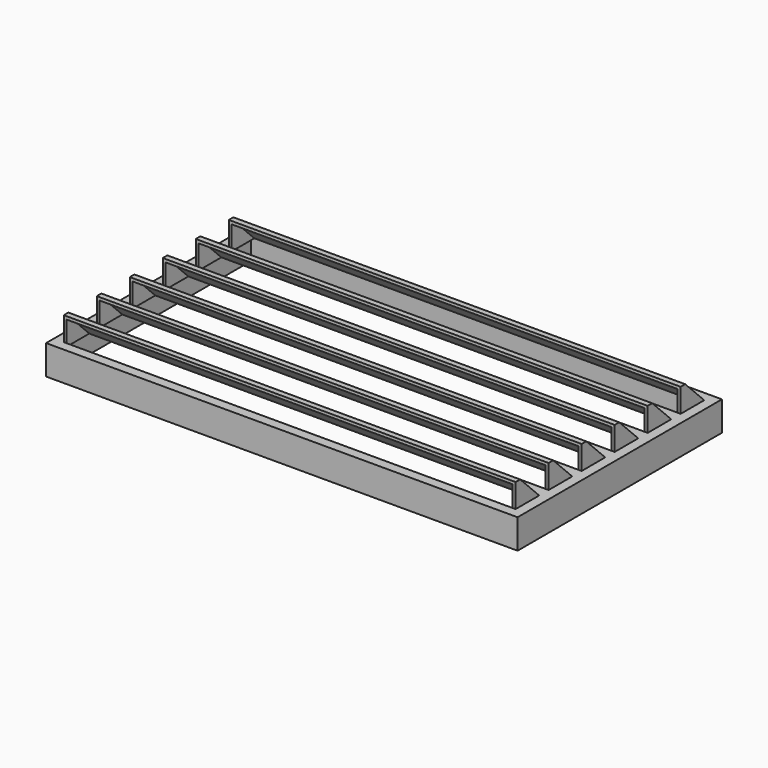
from build123d import *

# Parameters (mm, degrees)
F0_W         = 1200
F0_H         = 650
F1_DEPTH     = 75
F3_START     = -25
F3_DEPTH     = 1150
F4_T         = 7.5
F4_T3_DEPTH  = 90
F4_T5_DEPTH  = 1165
F4_T7_DEPTH  = 90
F4_T9_DEPTH  = 90
F4_T11_DEPTH = 90
F4_T13_DEPTH = 90
F4_T15_DEPTH = 90


# Not quite as in the source:
# - a shell that OpenCascade refuses in one call is made with other operations: the cavity is built on its own and cut out
# - a feature names something its author has since deleted; it is built from what else it names


with BuildPart() as f1:
    # F0 (on Top) → F1 (new body)
    with BuildSketch(Plane.XY):
        Rectangle(F0_W, F0_H)
    extrude(amount=F1_DEPTH)

    # F2 (on face) → F3 (join)
    with BuildSketch(Plane(origin=(-600, 0, 0), x_dir=(0, -1, 0), z_dir=(-1, 0, 0)).offset(F3_START)):
        Polygon((-239.4699645042, 135.5300354958), (-300, 75), (-225, 75), (-225, 135.5300354958), align=None)
        Polygon((-134.4699645042, 135.5300354958), (-195, 75), (-120, 75), (-120, 135.5300354958), align=None)
        Polygon((-29.4699645042, 135.5300354958), (-90, 75), (-15, 75), (-15, 135.5300354958), align=None)
        Polygon((75.5300354958, 135.5300354958), (15, 75), (90, 75), (90, 135.5300354958), align=None)
        Polygon((120, 75), (195, 75), (195, 135.5300354958), (180.5300354958, 135.5300354958), align=None)
        Polygon((225, 75), (300, 75), (300, 135.5300354958), (285.5300354958, 135.5300354958), align=None)
    extrude(amount=-F3_DEPTH)

    # F4: shell of thickness 7.5, made by hand


with BuildPart() as f4_core1:
    # F4_t2: copy of F1
    add(f1.part)

    # the walls: a layer under each face that stays
    f4_faces = [f4_core1.faces().sort_by_distance(p)[0] for p in [
        (0, -325, 37.5),
        (-600, 0, 37.5),
        (600, 0, 37.5),
        (0, 0, 75),
        (0, 325, 37.5),
        (-575, -262.5, 105.2650177479),
        (575, -262.5, 105.2650177479),
        (0, -255.2650177479, 105.2650177479),
        (-575, -157.5, 105.2650177479),
        (575, -157.5, 105.2650177479),
        (0, -150.2650177479, 105.2650177479),
        (-575, -52.5, 105.2650177479),
        (575, -52.5, 105.2650177479),
        (0, -45.2650177479, 105.2650177479),
        (-575, 52.5, 105.2650177479),
        (575, 52.5, 105.2650177479),
        (0, 59.7349822521, 105.2650177479),
        (-575, 157.5, 105.2650177479),
        (575, 157.5, 105.2650177479),
        (0, 164.7349822521, 105.2650177479),
        (-575, 262.5, 105.2650177479),
        (575, 262.5, 105.2650177479),
        (0, 269.7349822521, 105.2650177479),
        (0, -292.7650177479, 135.5300354958),
        (0, -187.7650177479, 135.5300354958),
        (0, -82.7650177479, 135.5300354958),
        (0, 22.2349822521, 135.5300354958),
        (0, 127.2349822521, 135.5300354958),
        (0, 232.2349822521, 135.5300354958),
    ]]
    thicken(f4_faces, amount=-F4_T, mode=Mode.SUBTRACT)

    # F4_s4 → F4_t3 (cut)
    with BuildSketch(Plane.XZ.offset(217.5)):
        Polygon((-575.075, 75.075), (-575, 67.5), (-567.5, 67.5), (-567.5, 75), align=None)
        Polygon((575.075, 75.075), (575, 67.5), (567.5, 67.5), (567.5, 75), align=None)
    extrude(amount=F4_T3_DEPTH, mode=Mode.SUBTRACT)

    # F4_s6 → F4_t5 (cut)
    with BuildSketch(Plane.YZ.offset(-582.5)):
        Polygon((-224.9469669914, 75.1280330086), (-225, 67.5), (-228.1066017178, 67.5), (-230.3033008589, 69.6966991411), align=None)
        Polygon((-119.9469669914, 75.1280330086), (-120, 67.5), (-123.1066017178, 67.5), (-125.3033008589, 69.6966991411), align=None)
        Polygon((-14.9469669914, 75.1280330086), (-15, 67.5), (-18.1066017178, 67.5), (-20.3033008589, 69.6966991411), align=None)
        Polygon((90.0530330086, 75.1280330086), (90, 67.5), (86.8933982822, 67.5), (84.6966991411, 69.6966991411), align=None)
        Polygon((195.0530330086, 75.1280330086), (195, 67.5), (191.8933982822, 67.5), (189.6966991411, 69.6966991411), align=None)
        Polygon((300.0530330086, 75.1280330086), (300, 67.5), (296.8933982822, 67.5), (294.6966991411, 69.6966991411), align=None)
    extrude(amount=F4_T5_DEPTH, mode=Mode.SUBTRACT)

    # F4_s8 → F4_t7 (cut)
    with BuildSketch(Plane.XZ.offset(112.5)):
        Polygon((-575.075, 75.075), (-575, 67.5), (-567.5, 67.5), (-567.5, 75), align=None)
        Polygon((575.075, 75.075), (575, 67.5), (567.5, 67.5), (567.5, 75), align=None)
    extrude(amount=F4_T7_DEPTH, mode=Mode.SUBTRACT)

    # F4_s10 → F4_t9 (cut)
    with BuildSketch(Plane.XZ.offset(7.5)):
        Polygon((-575.075, 75.075), (-575, 67.5), (-567.5, 67.5), (-567.5, 75), align=None)
        Polygon((575.075, 75.075), (575, 67.5), (567.5, 67.5), (567.5, 75), align=None)
    extrude(amount=F4_T9_DEPTH, mode=Mode.SUBTRACT)

    # F4_s12 → F4_t11 (cut)
    with BuildSketch(Plane.XZ.offset(-97.5)):
        Polygon((-575.075, 75.075), (-575, 67.5), (-567.5, 67.5), (-567.5, 75), align=None)
        Polygon((575.075, 75.075), (575, 67.5), (567.5, 67.5), (567.5, 75), align=None)
    extrude(amount=F4_T11_DEPTH, mode=Mode.SUBTRACT)

    # F4_s14 → F4_t13 (cut)
    with BuildSketch(Plane.XZ.offset(-202.5)):
        Polygon((-575.075, 75.075), (-575, 67.5), (-567.5, 67.5), (-567.5, 75), align=None)
        Polygon((575.075, 75.075), (575, 67.5), (567.5, 67.5), (567.5, 75), align=None)
    extrude(amount=F4_T13_DEPTH, mode=Mode.SUBTRACT)

    # F4_s16 → F4_t15 (cut)
    with BuildSketch(Plane.XZ.offset(-307.5)):
        Polygon((-575.075, 75.075), (-575, 67.5), (-567.5, 67.5), (-567.5, 75), align=None)
        Polygon((575.075, 75.075), (575, 67.5), (567.5, 67.5), (567.5, 75), align=None)
    extrude(amount=F4_T15_DEPTH, mode=Mode.SUBTRACT)


with BuildPart() as f1_1:
    add(f1.part)

    # what is left inside the walls is the cavity
    f4_cavity = [f4_core1.part.solids().sort_by_distance(p)[0] for p in [
        (0, -105.833333, 0.075),
    ]]
    add(f4_cavity, mode=Mode.SUBTRACT)


solid = f1_1.part
